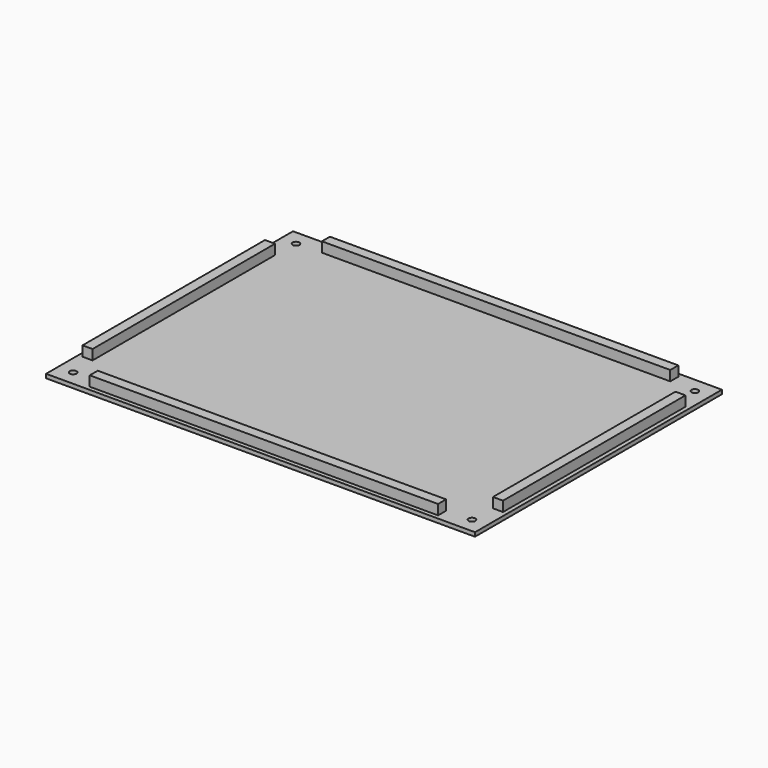
from build123d import *

# Parameters (mm, degrees)
F0_W     = 214
F0_H     = 154
F1_DEPTH = 2
F2_W     = 5
F2_H     = 113.8
F2_W_2   = 173.8
F2_H_2   = 5
F3_DEPTH = 5
F5_D     = 3.4
F5_DEPTH = 5
F5_TIP   = 1.0214630523


# Not quite as in the source:
# - a feature names something its author has since deleted; it is built from what else it names


with BuildPart() as f1:
    # F0 (on Top) → F1 (new body)
    with BuildSketch(Plane.XY):
        Rectangle(F0_W, F0_H)
    extrude(amount=F1_DEPTH)

    # F2 (on face) → F3 (join)
    with BuildSketch(Plane.XY.offset(2)):
        with Locations((-102.4, 0)):
            Rectangle(F2_W, F2_H)
        with Locations((0, 72.4)):
            Rectangle(F2_W_2, F2_H_2)
        with Locations((102.4, 0)):
            Rectangle(F2_W, F2_H)
        with Locations((0, -72.4)):
            Rectangle(F2_W_2, F2_H_2)
    extrude(amount=F3_DEPTH)

    # F5
    with Locations(Plane(origin=(0, 0, 0), x_dir=(1, 0, 0), z_dir=(0, 0, -1))):
        with Locations((-99.5, -69.5), (-99.5, 69.5), (99.5, 69.5), (99.5, -69.5)):
            Hole(F5_D / 2, depth=F5_DEPTH)
            with Locations((0, 0, -(F5_DEPTH + F5_TIP / 2))):  # 118° drill point
                Cone(0, F5_D / 2, F5_TIP, mode=Mode.SUBTRACT)


solid = f1.part
